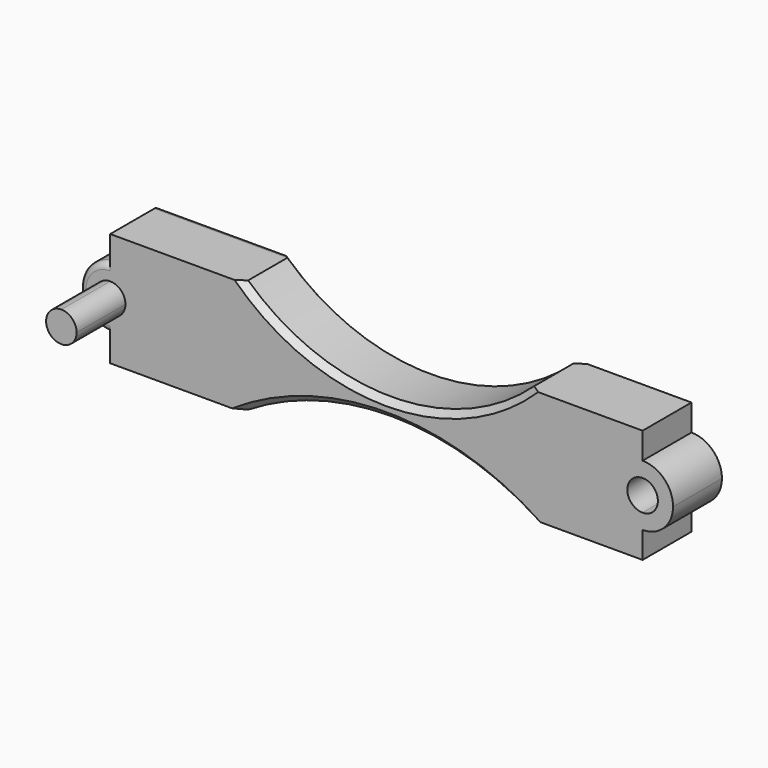
from build123d import *

# Parameters (mm, degrees)
F1_DEPTH = 50.8
F2_DEPTH = 50.8
F3_DEPTH = 25.4
F4_DEPTH = 101.6
F5_SIZE  = 5
F6_R     = 5


with BuildPart() as f1:
    # F0 (on Front) → F1 (new body)
    with BuildSketch(Plane.XZ):
        with BuildLine():
            Line((-81.5396818683, 48.140194267), (-192.2345156552, 48.140194267))
            Line((-192.2345156552, 48.140194267), (-192.2345156552, 26.0968099283))
            ThreePointArc((-192.2345156552, 26.0968099283), (-174.3603015656, 18.6930680356), (-166.956559673, 0.8188539461))
            ThreePointArc((-166.956559673, 0.8188539461), (-174.3603015656, -17.0553601435), (-192.2345156552, -24.4591020361))
            Line((-192.2345156552, -24.4591020361), (-192.2345156552, -46.5024863749))
            Line((-192.2345156552, -46.5024863749), (-81.5396818683, -46.5024863749))
            ThreePointArc((-81.5396818683, -46.5024863749), (37.4445138693, -12.4899673839), (156.4287096069, -46.5024863749))
            Line((156.4287096069, -46.5024863749), (250.5448194923, -46.5024863749))
            Line((250.5448194923, -46.5024863749), (250.5448194923, -24.5132009882))
            ThreePointArc((250.5448194923, -24.5132009882), (225.212764558, 0.8188539461), (250.5448194923, 26.1509088804))
            Line((250.5448194923, 26.1509088804), (250.5448194923, 48.140194267))
            Line((250.5448194923, 48.140194267), (156.4287096069, 48.140194267))
            ThreePointArc((156.4287096069, 48.140194267), (37.4445138693, 1.7154132922), (-81.5396818683, 48.140194267))
        make_face()
    extrude(amount=F1_DEPTH)

    # F0 (on Front) → F2 (join)
    with BuildSketch(Plane.XZ):
        with BuildLine():
            Line((-81.5396818683, 48.140194267), (-192.2345156552, 48.140194267))
            Line((-192.2345156552, 48.140194267), (-192.2345156552, 26.0968099283))
            ThreePointArc((-192.2345156552, 26.0968099283), (-174.3603015656, 18.6930680356), (-166.956559673, 0.8188539461))
            ThreePointArc((-166.956559673, 0.8188539461), (-174.3603015656, -17.0553601435), (-192.2345156552, -24.4591020361))
            Line((-192.2345156552, -24.4591020361), (-192.2345156552, -46.5024863749))
            Line((-192.2345156552, -46.5024863749), (-81.5396818683, -46.5024863749))
            ThreePointArc((-81.5396818683, -46.5024863749), (37.4445138693, -12.4899673839), (156.4287096069, -46.5024863749))
            Line((156.4287096069, -46.5024863749), (250.5448194923, -46.5024863749))
            Line((250.5448194923, -46.5024863749), (250.5448194923, -24.5132009882))
            ThreePointArc((250.5448194923, -24.5132009882), (225.212764558, 0.8188539461), (250.5448194923, 26.1509088804))
            Line((250.5448194923, 26.1509088804), (250.5448194923, 48.140194267))
            Line((250.5448194923, 48.140194267), (156.4287096069, 48.140194267))
            ThreePointArc((156.4287096069, 48.140194267), (37.4445138693, 1.7154132922), (-81.5396818683, 48.140194267))
        make_face()
        with BuildLine():
            ThreePointArc((-166.956559673, 0.8188539461), (-174.3603015656, 18.6930680356), (-192.2345156552, 26.0968099283))
            Line((-192.2345156552, 26.0968099283), (-192.2345156552, 13.5188539461))
            ThreePointArc((-192.2345156552, 13.5188539461), (-183.2542595341, 9.7991100672), (-179.5345156552, 0.8188539461))
            ThreePointArc((-179.5345156552, 0.8188539461), (-183.2542595341, -8.161402175), (-192.2345156552, -11.8811460539))
            Line((-192.2345156552, -11.8811460539), (-192.2345156552, -24.4591020361))
            ThreePointArc((-192.2345156552, -24.4591020361), (-174.3603015656, -17.0553601435), (-166.956559673, 0.8188539461))
        make_face()
        with BuildLine():
            Line((-192.2345156552, 13.5188539461), (-192.2345156552, 26.0968099283))
            ThreePointArc((-192.2345156552, 26.0968099283), (-217.5124716374, 0.8188539461), (-192.2345156552, -24.4591020361))
            Line((-192.2345156552, -24.4591020361), (-192.2345156552, -11.8811460539))
            ThreePointArc((-192.2345156552, -11.8811460539), (-204.9345156552, 0.8188539461), (-192.2345156552, 13.5188539461))
        make_face()
        with BuildLine():
            ThreePointArc((275.8768744265, 0.8188539461), (268.4572873177, 18.7313217715), (250.5448194923, 26.1509088804))
            Line((250.5448194923, 26.1509088804), (250.5448194923, 13.5188539461))
            ThreePointArc((250.5448194923, 13.5188539461), (259.5250756133, 9.7991100672), (263.2448194923, 0.8188539461))
            ThreePointArc((263.2448194923, 0.8188539461), (259.5250756133, -8.161402175), (250.5448194923, -11.8811460539))
            Line((250.5448194923, -11.8811460539), (250.5448194923, -24.5132009882))
            ThreePointArc((250.5448194923, -24.5132009882), (268.4572873177, -17.0936138793), (275.8768744265, 0.8188539461))
        make_face()
        with BuildLine():
            Line((250.5448194923, 13.5188539461), (250.5448194923, 26.1509088804))
            ThreePointArc((250.5448194923, 26.1509088804), (225.212764558, 0.8188539461), (250.5448194923, -24.5132009882))
            Line((250.5448194923, -24.5132009882), (250.5448194923, -11.8811460539))
            ThreePointArc((250.5448194923, -11.8811460539), (237.8448194923, 0.8188539461), (250.5448194923, 13.5188539461))
        make_face()
    extrude(amount=F2_DEPTH)

    # F0 (on Front) → F3 (join)
    with BuildSketch(Plane.XZ):
        with BuildLine():
            Line((-81.5396818683, 48.140194267), (-192.2345156552, 48.140194267))
            Line((-192.2345156552, 48.140194267), (-192.2345156552, 26.0968099283))
            ThreePointArc((-192.2345156552, 26.0968099283), (-174.3603015656, 18.6930680356), (-166.956559673, 0.8188539461))
            ThreePointArc((-166.956559673, 0.8188539461), (-174.3603015656, -17.0553601435), (-192.2345156552, -24.4591020361))
            Line((-192.2345156552, -24.4591020361), (-192.2345156552, -46.5024863749))
            Line((-192.2345156552, -46.5024863749), (-81.5396818683, -46.5024863749))
            ThreePointArc((-81.5396818683, -46.5024863749), (37.4445138693, -12.4899673839), (156.4287096069, -46.5024863749))
            Line((156.4287096069, -46.5024863749), (250.5448194923, -46.5024863749))
            Line((250.5448194923, -46.5024863749), (250.5448194923, -24.5132009882))
            ThreePointArc((250.5448194923, -24.5132009882), (225.212764558, 0.8188539461), (250.5448194923, 26.1509088804))
            Line((250.5448194923, 26.1509088804), (250.5448194923, 48.140194267))
            Line((250.5448194923, 48.140194267), (156.4287096069, 48.140194267))
            ThreePointArc((156.4287096069, 48.140194267), (37.4445138693, 1.7154132922), (-81.5396818683, 48.140194267))
        make_face()
        with BuildLine():
            ThreePointArc((-166.956559673, 0.8188539461), (-174.3603015656, 18.6930680356), (-192.2345156552, 26.0968099283))
            Line((-192.2345156552, 26.0968099283), (-192.2345156552, 13.5188539461))
            ThreePointArc((-192.2345156552, 13.5188539461), (-183.2542595341, 9.7991100672), (-179.5345156552, 0.8188539461))
            ThreePointArc((-179.5345156552, 0.8188539461), (-183.2542595341, -8.161402175), (-192.2345156552, -11.8811460539))
            Line((-192.2345156552, -11.8811460539), (-192.2345156552, -24.4591020361))
            ThreePointArc((-192.2345156552, -24.4591020361), (-174.3603015656, -17.0553601435), (-166.956559673, 0.8188539461))
        make_face()
        with BuildLine():
            Line((-192.2345156552, 13.5188539461), (-192.2345156552, 26.0968099283))
            ThreePointArc((-192.2345156552, 26.0968099283), (-217.5124716374, 0.8188539461), (-192.2345156552, -24.4591020361))
            Line((-192.2345156552, -24.4591020361), (-192.2345156552, -11.8811460539))
            ThreePointArc((-192.2345156552, -11.8811460539), (-204.9345156552, 0.8188539461), (-192.2345156552, 13.5188539461))
        make_face()
        with BuildLine():
            ThreePointArc((275.8768744265, 0.8188539461), (268.4572873177, 18.7313217715), (250.5448194923, 26.1509088804))
            Line((250.5448194923, 26.1509088804), (250.5448194923, 13.5188539461))
            ThreePointArc((250.5448194923, 13.5188539461), (259.5250756133, 9.7991100672), (263.2448194923, 0.8188539461))
            ThreePointArc((263.2448194923, 0.8188539461), (259.5250756133, -8.161402175), (250.5448194923, -11.8811460539))
            Line((250.5448194923, -11.8811460539), (250.5448194923, -24.5132009882))
            ThreePointArc((250.5448194923, -24.5132009882), (268.4572873177, -17.0936138793), (275.8768744265, 0.8188539461))
        make_face()
        with BuildLine():
            Line((250.5448194923, 13.5188539461), (250.5448194923, 26.1509088804))
            ThreePointArc((250.5448194923, 26.1509088804), (225.212764558, 0.8188539461), (250.5448194923, -24.5132009882))
            Line((250.5448194923, -24.5132009882), (250.5448194923, -11.8811460539))
            ThreePointArc((250.5448194923, -11.8811460539), (237.8448194923, 0.8188539461), (250.5448194923, 13.5188539461))
        make_face()
    extrude(amount=F3_DEPTH)

    # F0 (on Front) → F4 (join)
    with BuildSketch(Plane.XZ):
        with BuildLine():
            ThreePointArc((-179.5345156552, 0.8188539461), (-183.2542595341, 9.7991100672), (-192.2345156552, 13.5188539461))
            ThreePointArc((-192.2345156552, 13.5188539461), (-204.9345156552, 0.8188539461), (-192.2345156552, -11.8811460539))
            ThreePointArc((-192.2345156552, -11.8811460539), (-183.2542595341, -8.161402175), (-179.5345156552, 0.8188539461))
        make_face()
    extrude(amount=F4_DEPTH)

    # F5
    f5_edges = [f1.edges().sort_by_distance(p)[0] for p in [
        (37.444514, 0, 1.715413),
        (37.444514, 0, -12.489967),
        (37.444514, -50.8, 1.715413),
        (37.444514, -50.8, -12.489967),
    ]]
    chamfer(f5_edges, length=F5_SIZE)

    # F6
    f6_edges = [f1.edges().sort_by_distance(p)[0] for p in [
        (-140.520101, 0, 48.140194),
        (-217.512472, 0, 0.818854),
        (-217.512472, -50.8, 0.818854),
    ]]
    fillet(f6_edges, radius=F6_R)


solid = f1.part
